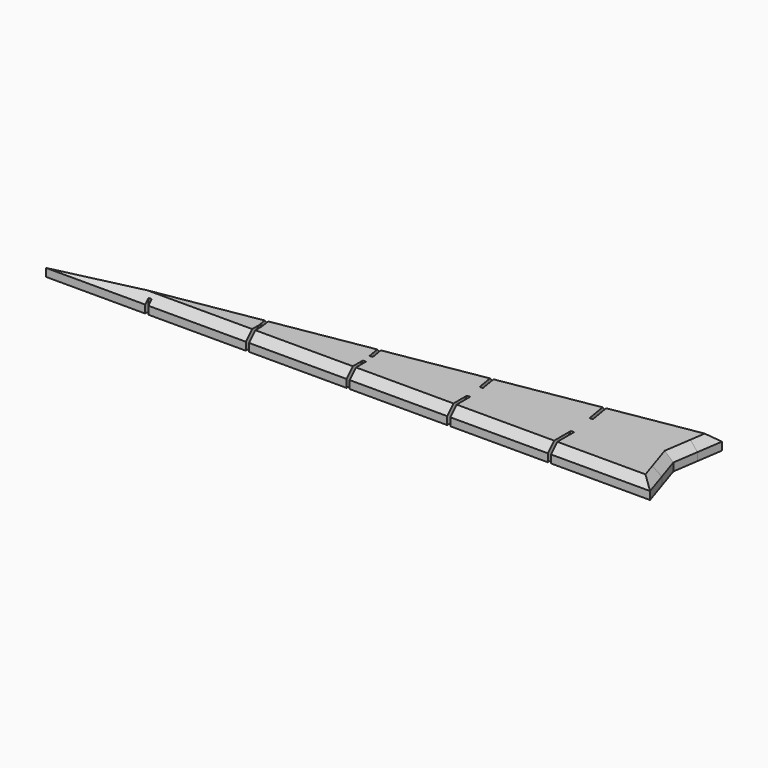
from build123d import *

# Parameters (mm, degrees)
F2_DEPTH    = 4
F3_C1_SIZE  = 2
F3_C2_SIZE  = 2
F3_C3_SIZE  = 2
F3_C4_SIZE  = 2
F3_C5_SIZE  = 2
F3_C6_SIZE  = 2
F3_C7_SIZE  = 2
F3_C8_SIZE  = 2
F3_C9_SIZE  = 2
F3_C10_SIZE = 2


with BuildPart() as f2:
    # F1 (on Top) → F2 (new body)
    with BuildSketch(Plane.XY):
        Polygon((-25, 0), (0, 0), (-2.0441389628, 6.2647895141), (-25, 5.3083011104), align=None)
        Polygon((-25, 5.3083011104), (-2.0441389628, 6.2647895141), (-4.0478985191, 12.4058259531), (-75.8, 6.4056137967), (-75.8, 3.1916472924), (-51.2, 4.2166410704), (-51.2, 7.6929950155), (-50.4, 7.6929950155), (-50.4, 4.2499742014), (-25.8, 5.2749679794), (-25.8, 7.6929950155), (-25, 7.6929950155), align=None)
        Polygon((-50.4, 0), (-25.8, 0), (-25.8, 5.2749679794), (-50.4, 4.2499742014), align=None)
        Polygon((-75.8, 0), (-51.2, 0), (-51.2, 4.2166410704), (-75.8, 3.1916472924), align=None)
        Polygon((-51.2, 4.2166410704), (-50.4, 4.2499742014), (-50.4, 7.6929950155), (-51.2, 7.6929950155), align=None)
        Polygon((-25.8, 5.2749679794), (-25, 5.3083011104), (-25, 7.6929950155), (-25.8, 7.6929950155), align=None)
        Polygon((-76.6, 3.1583141614), (-76.6, 6.3387144359), (-101.2, 4.2815590912), (-101.2, 2.1333203834), align=None)
        Polygon((-75.8, 3.1916472924), (-75.8, 6.4056137967), (-76.6, 6.3387144359), (-76.6, 3.1583141614), align=None)
        Polygon((-76.6, 0), (-76.6, 3.1583141614), (-101.2, 2.1333203834), (-101.2, 0), align=None)
        Polygon((-101.2, 2.1333203834), (-101.2, 4.2815590912), (-102, 4.2146597304), (-102, 2.0999872524), align=None)
        Polygon((-102, 0), (-102, 2.0999872524), (-126.6, 1.0749934745), (-126.6, 0), align=None)
        Polygon((-102, 2.0999872524), (-102, 4.2146597304), (-126.6, 2.1575043858), (-126.6, 1.0749934745), align=None)
        Polygon((-126.6, 1.0749934745), (-126.6, 2.1575043858), (-127.4, 2.090605025), (-127.4, 1.0416603435), align=None)
        Polygon((-127.4, 1.0416603435), (-127.4, 2.090605025), (-152.4, 0), align=None)
        Polygon((-127.4, 1.0416603435), (-152.4, 0), (-127.4, 0), align=None)
    extrude(amount=F2_DEPTH)

    # F3: chamfer of 2 on 11 edges, made by hand

    # F3_c1
    f3_c1_edges = [f2.edges().sort_by_distance(p)[0] for p in [
        (-12.5, 0, 4),
    ]]
    chamfer(f3_c1_edges, length=F3_C1_SIZE)

    # F3_c2
    f3_c2_edges = [f2.edges().sort_by_distance(p)[0] for p in [
        (-2.350239386, 7.2029129766, 4),
    ]]
    chamfer(f3_c2_edges, length=F3_C2_SIZE)

    # F3_c3
    f3_c3_edges = [f2.edges().sort_by_distance(p)[0] for p in [
        (-139.9, 0, 4),
    ]]
    chamfer(f3_c3_edges, length=F3_C3_SIZE)

    # F3_c4
    f3_c4_edges = [f2.edges().sort_by_distance(p)[0] for p in [
        (-101.6, 2.1166538179, 4),
    ]]
    chamfer(f3_c4_edges, length=F3_C4_SIZE)

    # F3_c5
    f3_c5_edges = [f2.edges().sort_by_distance(p)[0] for p in [
        (-88.9, 0, 4),
    ]]
    chamfer(f3_c5_edges, length=F3_C5_SIZE)

    # F3_c6
    f3_c6_edges = [f2.edges().sort_by_distance(p)[0] for p in [
        (-76.2, 3.1749807269, 4),
    ]]
    chamfer(f3_c6_edges, length=F3_C6_SIZE)

    # F3_c7
    f3_c7_edges = [f2.edges().sort_by_distance(p)[0] for p in [
        (-63.5, 0, 4),
    ]]
    chamfer(f3_c7_edges, length=F3_C7_SIZE)

    # F3_c8
    f3_c8_edges = [f2.edges().sort_by_distance(p)[0] for p in [
        (-50.8, 4.2333076359, 4),
    ]]
    chamfer(f3_c8_edges, length=F3_C8_SIZE)

    # F3_c9
    f3_c9_edges = [f2.edges().sort_by_distance(p)[0] for p in [
        (-38.1, 0, 4),
    ]]
    chamfer(f3_c9_edges, length=F3_C9_SIZE)

    # F3_c10
    f3_c10_edges = [f2.edges().sort_by_distance(p)[0] for p in [
        (-25.4, 5.2916345449, 4),
    ]]
    chamfer(f3_c10_edges, length=F3_C10_SIZE)

    # F4: F2 across face


with BuildPart() as f2_1:
    add(f2.part)
    add(f2.part.mirror(Plane(origin=(-75.6988371999, 6.414073455, 1.938990945), x_dir=(-0.9965217286, -0.0833333333, 0), z_dir=(-0.0833333333, 0.9965217286, 0))))


solid = f2_1.part
